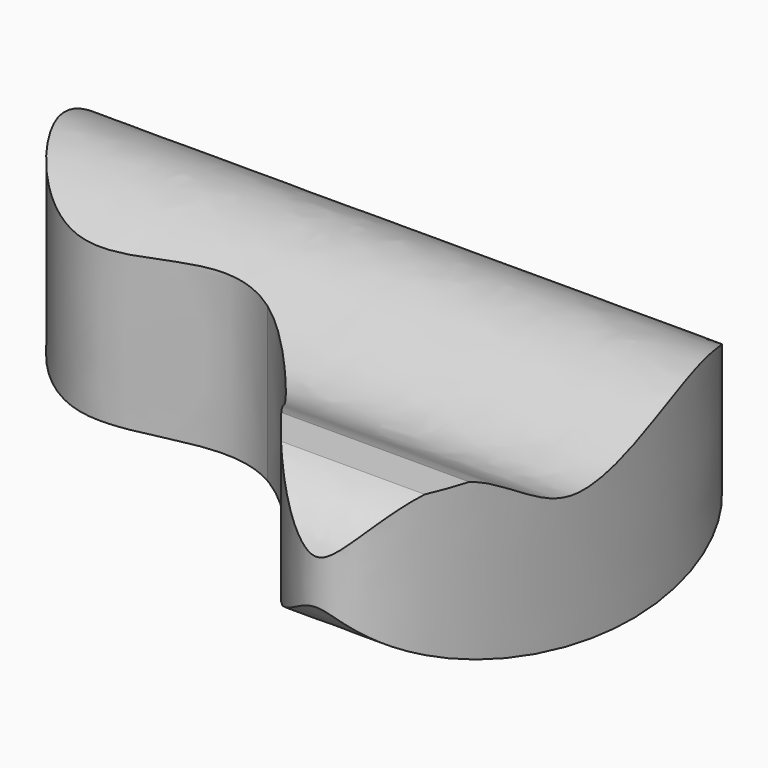
from build123d import *

# Parameters (mm, degrees)
F1_DEPTH = 30
F3_START = -56
F3_DEPTH = 124


# Not quite as in the source:
# - a feature of the source that left no trace in its solid (it failed there, or was rolled back) is left out


with BuildPart() as f1:
    # F0 (on Top) → F1 (new body)
    with BuildSketch(Plane.XY):
        with BuildLine():
            add(Edge.make_bspline(
                [(0, 0), (15.7172503683, -8.911807573), (51.8188373943, -90.1440382977), (72.8520047816, 54.107021769), (-3.8603481253, 16.9825139076), (-26.8793414158, 53.5768472549), (-60.0530534094, 29.2808657148), (-31.2913550395, -11.2245511197), (-10.8537106561, 6.1541413768), (0, 0)],
                knots=[0, 0, 0, 0, 0.1742938346, 0.3577270692, 0.5173926964, 0.6431092334, 0.7530442247, 0.8796395803, 1, 1, 1, 1], degree=3))
        make_face()
    extrude(amount=F1_DEPTH)

    # F2 (on Right) → F3 (intersect)
    with BuildSketch(Plane.YZ.offset(F3_START)):
        with BuildLine():
            add(Edge.make_bspline(
                [(-46.1890548468, 17.0933511108), (-47.0858050751, 23.2020363459), (-30.8616926385, 37.827425399), (-12.855477351, 13.9463688607), (16.5141982701, 38.1330111818), (45.7245120632, 10.029141404), (0.065487853, -6.4036129617), (-44.7482673433, 7.2786701978), (-46.1890548468, 17.0933511108)],
                knots=[0, 0, 0, 0, 0.1345596823, 0.2782981281, 0.4489816972, 0.5964074946, 0.7838061228, 1, 1, 1, 1], degree=3))
        make_face()
    extrude(amount=F3_DEPTH, mode=Mode.INTERSECT)


solid = f1.part
